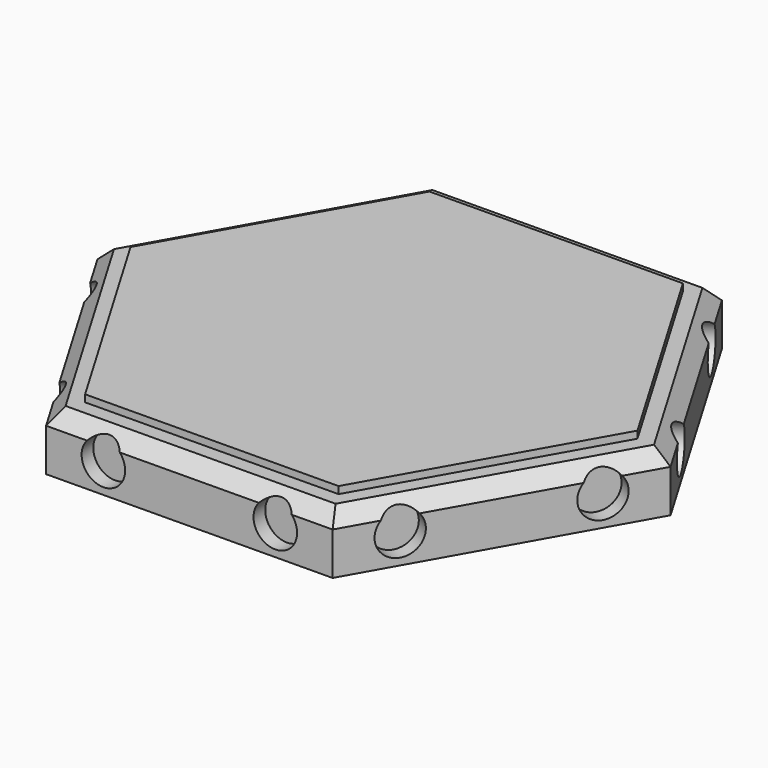
from build123d import *

# Parameters (mm, degrees)
F1_DEPTH      = 4.5
F2_DEPTH      = 4
F3_T          = -2.5
F4_R          = 1.52
F5_DEPTH      = 1.04
F6_R          = 1.52
F7_DEPTH      = 1.04
F8_R          = 1.52
F9_DEPTH      = 1.04
F10_R         = 1.52
F11_DEPTH     = 1.04
F12_R         = 1.52
F13_DEPTH     = 1.04
F14_R         = 1.52
F15_DEPTH     = 1.04
F16_T1_DEPTH  = 25.1433659759
F16_T3_DEPTH  = 25.1433659759
F16_T5_DEPTH  = 25.1433659759
F16_T7_DEPTH  = 25.1433659759
F16_T9_DEPTH  = 25.1433659759
F16_T11_DEPTH = 25.1433659759


# Not quite as in the source:
# - a fillet or chamfer that OpenCascade refuses, or shapes differently, is made with other operations: its cross-section is extruded or revolved along the edge and cut away or added


with BuildPart() as f1:
    # F0 (on Top) → F1 (new body)
    with BuildSketch(Plane.XY):
        Polygon((-8.9919036831, 15.2349256124), (-17.6897844467, -0.1697542118), (-8.6978807636, -15.4046798242), (8.9919036831, -15.2349256124), (17.6897844467, 0.1697542118), (8.6978807636, 15.4046798242), align=None)
    extrude(amount=F1_DEPTH)

    # F0 (on Top) → F2 (join)
    with BuildSketch(Plane.XY):
        Polygon((-19.9990791985, -0.1919146011), (-9.8333366793, -17.4156679387), (10.1657425191, -17.2237533376), (19.9990791985, 0.1919146011), (9.8333366793, 17.4156679387), (-10.1657425191, 17.2237533376), align=None)
        Polygon((-8.6978807636, -15.4046798242), (-17.6897844467, -0.1697542118), (-8.9919036831, 15.2349256124), (8.6978807636, 15.4046798242), (17.6897844467, 0.1697542118), (8.9919036831, -15.2349256124), align=None, mode=Mode.SUBTRACT)
    extrude(amount=F2_DEPTH)

    # F3
    f3_openings = [f1.faces().sort_by_distance(p)[0] for p in [
        (0, 0, 0),
    ]]
    offset(amount=F3_T, openings=f3_openings, kind=Kind.INTERSECTION)

    # F4 (on face) → F5 (cut)
    with BuildSketch(Plane(origin=(15.0824108588, -8.5159193683, 0), x_dir=(0.491666834, 0.8707833969, 0), z_dir=(0.8707833969, -0.491666834, 0))):
        with Locations((-6, 2)):
            Circle(F4_R)
        with Locations((6, 2)):
            Circle(F4_R)
    extrude(amount=-F5_DEPTH, mode=Mode.SUBTRACT)

    # F6 (on face) → F7 (cut)
    with BuildSketch(Plane(origin=(0.1662029199, -17.3197106382, 0), x_dir=(0.9999539599, 0.0095957301, 0), z_dir=(0.0095957301, -0.9999539599, 0))):
        with Locations((-6, 2)):
            Circle(F6_R)
        with Locations((6, 2)):
            Circle(F6_R)
    extrude(amount=-F7_DEPTH, mode=Mode.SUBTRACT)

    # F8 (on face) → F9 (cut)
    with BuildSketch(Plane(origin=(-14.9162079389, -8.8037912699, 0), x_dir=(0.508287126, -0.8611876669, 0), z_dir=(-0.8611876669, -0.508287126, 0))):
        with Locations((-6, 2)):
            Circle(F8_R)
        with Locations((6, 2)):
            Circle(F8_R)
    extrude(amount=-F9_DEPTH, mode=Mode.SUBTRACT)

    # F10 (on face) → F11 (cut)
    with BuildSketch(Plane(origin=(-15.0824108588, 8.5159193683, 0), x_dir=(-0.491666834, -0.8707833969, 0), z_dir=(-0.8707833969, 0.491666834, 0))):
        with Locations((-6, 2)):
            Circle(F10_R)
        with Locations((6, 2)):
            Circle(F10_R)
    extrude(amount=-F11_DEPTH, mode=Mode.SUBTRACT)

    # F12 (on face) → F13 (cut)
    with BuildSketch(Plane(origin=(-0.1662029199, 17.3197106382, 0), x_dir=(-0.9999539599, -0.0095957301, 0), z_dir=(-0.0095957301, 0.9999539599, 0))):
        with Locations((-6, 2)):
            Circle(F12_R)
        with Locations((6, 2)):
            Circle(F12_R)
    extrude(amount=-F13_DEPTH, mode=Mode.SUBTRACT)

    # F14 (on face) → F15 (cut)
    with BuildSketch(Plane(origin=(14.9162079389, 8.8037912699, 0), x_dir=(-0.508287126, 0.8611876669, 0), z_dir=(0.8611876669, 0.508287126, 0))):
        with Locations((-6, 2)):
            Circle(F14_R)
        with Locations((6, 2)):
            Circle(F14_R)
    extrude(amount=-F15_DEPTH, mode=Mode.SUBTRACT)

    # F16: chamfer of 1 on 6 edges, made by hand

    # F16_s2 → F16_t1 (cut)
    with BuildSketch(Plane(origin=(6.3900246144, -10.8265783412, 0), x_dir=(0, 0, 1), z_dir=(-0.508287126, 0.8611876669, 0))):
        Polygon((4, 16.3205080757), (3, 17.3205080757), (4, 17.3205080757), align=None)
    extrude(amount=F16_T1_DEPTH, mode=Mode.SUBTRACT)

    # F16_s4 → F16_t3 (cut)
    with BuildSketch(Plane(origin=(-6.1810795723, -10.9472128174, 0), x_dir=(0, 0, 1), z_dir=(0.491666834, 0.8707833969, 0))):
        Polygon((4, 16.3205080757), (3, 17.3205080757), (4, 17.3205080757), align=None)
    extrude(amount=F16_T3_DEPTH, mode=Mode.SUBTRACT)

    # F16_s6 → F16_t5 (cut)
    with BuildSketch(Plane(origin=(-12.5711041867, -0.1206344763, 0), x_dir=(0, 0, 1), z_dir=(0.9999539599, 0.0095957301, 0))):
        Polygon((4, 16.3205080757), (3, 17.3205080757), (4, 17.3205080757), align=None)
    extrude(amount=F16_T5_DEPTH, mode=Mode.SUBTRACT)

    # F16_s8 → F16_t7 (cut)
    with BuildSketch(Plane(origin=(-6.3900246144, 10.8265783412, 0), x_dir=(0, 0, 1), z_dir=(0.508287126, -0.8611876669, 0))):
        Polygon((4, 16.3205080757), (3, 17.3205080757), (4, 17.3205080757), align=None)
    extrude(amount=F16_T7_DEPTH, mode=Mode.SUBTRACT)

    # F16_s10 → F16_t9 (cut)
    with BuildSketch(Plane(origin=(6.1810795723, 10.9472128174, 0), x_dir=(0, 0, 1), z_dir=(-0.491666834, -0.8707833969, 0))):
        Polygon((4, 16.3205080757), (3, 17.3205080757), (4, 17.3205080757), align=None)
    extrude(amount=F16_T9_DEPTH, mode=Mode.SUBTRACT)

    # F16_s12 → F16_t11 (cut)
    with BuildSketch(Plane(origin=(12.5711041867, 0.1206344763, 0), x_dir=(0, 0, 1), z_dir=(-0.9999539599, -0.0095957301, 0))):
        Polygon((4, 16.3205080757), (3, 17.3205080757), (4, 17.3205080757), align=None)
    extrude(amount=F16_T11_DEPTH, mode=Mode.SUBTRACT)


solid = f1.part
